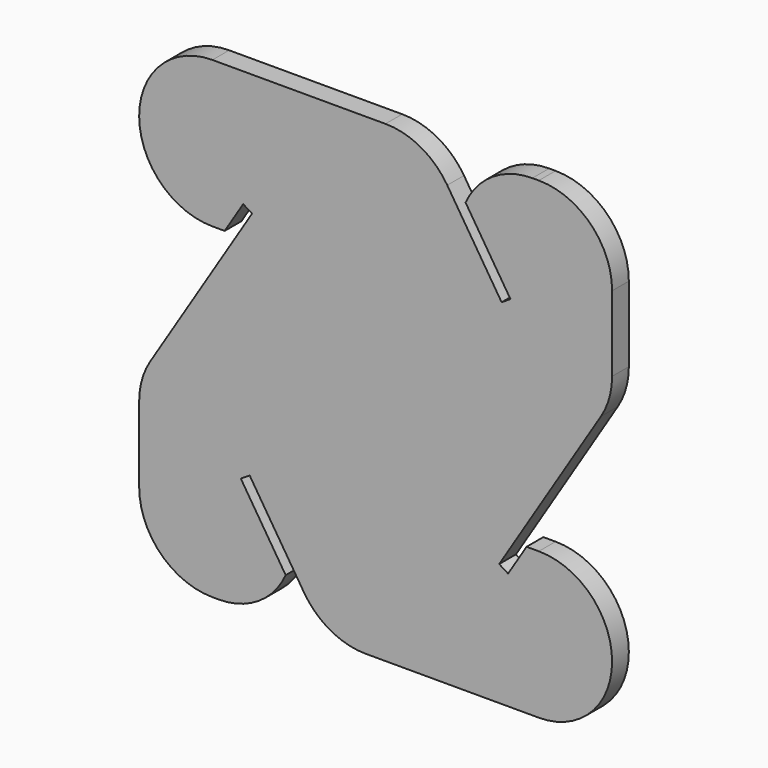
from build123d import *

# Parameters (mm, degrees)
F1_DEPTH     = 100
F2_T1_DEPTH  = 1850
F2_T3_DEPTH  = 1695.9707417334
F2_T5_DEPTH  = 1695.9706144549
F2_T7_DEPTH  = 601.1121280065
F2_T9_DEPTH  = 1060.1512237757
F2_T11_DEPTH = 601.1120863274
F2_T13_DEPTH = 1060.1510758761


# Not quite as in the source:
# - a fillet or chamfer that OpenCascade refuses, or shapes differently, is made with other operations: its cross-section is extruded or revolved along the edge and cut away or added


with BuildPart() as f1:
    # F0 (on Front) → F1 (new body)
    with BuildSketch(Plane.XZ):
        Polygon((1129.7543572, 319.6687281531), (1129.7543572, 1129.7543953), (429.7543572, 1129.7543953), (429.7543572, 923.3339748412), (644.069888311, 586.8814977509), (601.898706638, 560.0190437248), (238.9852410529, 1129.7543953), (-1129.7543572, 1129.7543953), (-1129.7543572, 429.7543953), (-721.1567962335, 429.7543953), (-632.764270148, 571.4424256952), (-590.342503852, 544.9774725622), (-1129.7543572, -319.6680631783), (-1129.7543572, -1129.7543953), (-429.7543572, -1129.7543953), (-429.7543572, -923.3340314322), (-644.0698939815, -586.8814489736), (-601.8987088185, -560.0190004264), (-238.9853197059, -1129.7543953), (1129.7543572, -1129.7543953), (1129.7543572, -429.7543953), (721.156425601, -429.7543953), (632.7643072985, -571.4417859327), (590.3425398375, -544.9768346673), align=None)
    extrude(amount=F1_DEPTH)

    # F2: fillet of radius 350 on 12 edges, made by hand

    # F2_s2 → F2_t1 (cut)
    with BuildSketch(Plane.XZ.offset(-875)):
        with BuildLine():
            ThreePointArc((1129.7543572, 779.7543953), (1027.2417306153, 1027.2417687153), (779.7543572, 1129.7543953))
            Line((779.7543572, 1129.7543953), (1129.7543572, 1129.7543953))
            Line((1129.7543572, 1129.7543953), (1129.7543572, 779.7543953))
        make_face()
        with BuildLine():
            ThreePointArc((-779.7543572, 1129.7543953), (-1027.2417306153, 1027.2417687153), (-1129.7543572, 779.7543953))
            Line((-1129.7543572, 779.7543953), (-1129.7543572, 1129.7543953))
            Line((-1129.7543572, 1129.7543953), (-779.7543572, 1129.7543953))
        make_face()
        with BuildLine():
            ThreePointArc((-1129.7543572, 779.7543953), (-1027.2417306153, 532.2670218847), (-779.7543572, 429.7543953))
            Line((-779.7543572, 429.7543953), (-1129.7543572, 429.7543953))
            Line((-1129.7543572, 429.7543953), (-1129.7543572, 779.7543953))
        make_face()
        with BuildLine():
            ThreePointArc((-1129.7543572, -779.7543953), (-1027.2417306153, -1027.2417687153), (-779.7543572, -1129.7543953))
            Line((-779.7543572, -1129.7543953), (-1129.7543572, -1129.7543953))
            Line((-1129.7543572, -1129.7543953), (-1129.7543572, -779.7543953))
        make_face()
        with BuildLine():
            ThreePointArc((1129.7543572, -779.7543953), (1027.2417306153, -1027.2417687153), (779.7543572, -1129.7543953))
            Line((779.7543572, -1129.7543953), (1129.7543572, -1129.7543953))
            Line((1129.7543572, -1129.7543953), (1129.7543572, -779.7543953))
        make_face()
        with BuildLine():
            ThreePointArc((1129.7543572, -779.7543953), (1027.2417306153, -532.2670218847), (779.7543572, -429.7543953))
            Line((779.7543572, -429.7543953), (1129.7543572, -429.7543953))
            Line((1129.7543572, -429.7543953), (1129.7543572, -779.7543953))
        make_face()
    extrude(amount=F2_T1_DEPTH, mode=Mode.SUBTRACT)

    # F2_s4 → F2_t3 (cut)
    with BuildSketch(Plane.XZ.offset(-797.9853708667)):
        with BuildLine():
            ThreePointArc((748.9485055467, 1129.7543953), (558.8864799332, 1073.653062224), (429.7543572, 923.3339748412))
            Line((429.7543572, 923.3339748412), (429.7543572, 1129.7543953))
            Line((429.7543572, 1129.7543953), (748.9485055467, 1129.7543953))
        make_face()
    extrude(amount=F2_T3_DEPTH, mode=Mode.SUBTRACT)

    # F2_s6 → F2_t5 (cut)
    with BuildSketch(Plane.XZ.offset(-797.9853072275)):
        with BuildLine():
            ThreePointArc((-748.948480091, -1129.7543953), (-558.8864805307, -1073.6530790724), (-429.7543572, -923.3340314322))
            Line((-429.7543572, -923.3340314322), (-429.7543572, -1129.7543953))
            Line((-429.7543572, -1129.7543953), (-748.948480091, -1129.7543953))
        make_face()
    extrude(amount=F2_T5_DEPTH, mode=Mode.SUBTRACT)

    # F2_s8 → F2_t7 (cut)
    with BuildSketch(Plane.XZ.offset(-250.5560640033)):
        with BuildLine():
            ThreePointArc((-1076.7067212718, -234.6358168488), (-1116.2311969863, -323.5404172309), (-1129.7543572, -419.8904887796))
            Line((-1129.7543572, -419.8904887796), (-1129.7543572, -319.6680631783))
            Line((-1129.7543572, -319.6680631783), (-1076.7067212718, -234.6358168488))
        make_face()
    extrude(amount=F2_T7_DEPTH, mode=Mode.SUBTRACT)

    # F2_s10 → F2_t9 (cut)
    with BuildSketch(Plane.XZ.offset(-480.0756118878)):
        with BuildLine():
            ThreePointArc((-342.1533710911, -967.7915351311), (-215.310355621, -1086.6037059892), (-46.9550749508, -1129.7543953))
            Line((-46.9550749508, -1129.7543953), (-238.9853197059, -1129.7543953))
            Line((-238.9853197059, -1129.7543953), (-342.1533710911, -967.7915351311))
        make_face()
    extrude(amount=F2_T9_DEPTH, mode=Mode.SUBTRACT)

    # F2_s12 → F2_t11 (cut)
    with BuildSketch(Plane.XZ.offset(-250.5560431637)):
        with BuildLine():
            ThreePointArc((1076.7067294274, 234.6364865607), (1116.2311991071, 323.5410812763), (1129.7543572, 419.8911454186))
            Line((1129.7543572, 419.8911454186), (1129.7543572, 319.6687281531))
            Line((1129.7543572, 319.6687281531), (1076.7067294274, 234.6364865607))
        make_face()
    extrude(amount=F2_T11_DEPTH, mode=Mode.SUBTRACT)

    # F2_s14 → F2_t13 (cut)
    with BuildSketch(Plane.XZ.offset(-480.0755379381)):
        with BuildLine():
            ThreePointArc((342.1532975884, 967.791573483), (215.3102866151, 1086.6037169255), (46.9550258777, 1129.7543953))
            Line((46.9550258777, 1129.7543953), (238.9852410529, 1129.7543953))
            Line((238.9852410529, 1129.7543953), (342.1532975884, 967.791573483))
        make_face()
    extrude(amount=F2_T13_DEPTH, mode=Mode.SUBTRACT)


solid = f1.part
